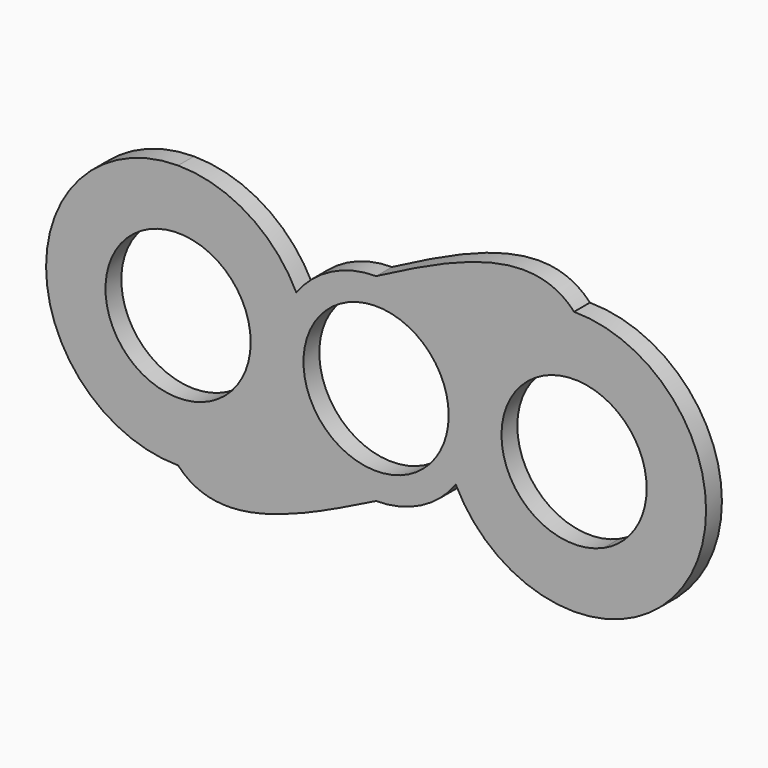
from build123d import *

# Parameters (mm, degrees)
F0_R     = 11
F1_DEPTH = 3


with BuildPart() as f1:
    # F0 (on Front) → F1 (new body)
    with BuildSketch(Plane.XZ):
        with BuildLine():
            ThreePointArc((34.4457053252, 10.0615955075), (39.2169072518, 6.0040503586), (41, -2e-10))
            ThreePointArc((41, -2e-10), (39.218122302, -6.0021847046), (34.4497779591, -10.0597950337))
            add(Edge.make_bspline(
                [(34.4497779591, -10.0597950337), (33.5572864984, -14.2139641421), (32.0732731389, -17.7845741491), (30, -20)],
                knots=[0.5781750695, 0.5781750695, 0.5781750695, 0.5781750695, 0.6822186894, 0.6822186894, 0.6822186894, 0.6822186894], degree=3))
            ThreePointArc((30, -20), (50, 0), (30, 20))
            add(Edge.make_bspline(
                [(30, 20), (32.0727475467, 17.7685869814), (33.5539058525, 14.2021827738), (34.4457053252, 10.0615955075)],
                knots=[0.3177813106, 0.3177813106, 0.3177813106, 0.3177813106, 0.4213364669, 0.4213364669, 0.4213364669, 0.4213364669], degree=3))
        make_face()
        with BuildLine():
            ThreePointArc((34.4497779591, -10.0597950337), (19.0000002253, -0.0022264354), (34.4457053252, 10.0615955075))
            add(Edge.make_bspline(
                [(30, 20), (32.0727475467, 17.7685869814), (33.5539058525, 14.2021827738), (34.4457053252, 10.0615955075)],
                knots=[0.3177813106, 0.3177813106, 0.3177813106, 0.3177813106, 0.4213364669, 0.4213364669, 0.4213364669, 0.4213364669], degree=3))
            add(Edge.make_bspline(
                [(0, 15), (11.7076504976, 21.1235117167), (23.6393275279, 26.8475716609), (30, 20)],
                knots=[0, 0, 0, 0, 0.3177813106, 0.3177813106, 0.3177813106, 0.3177813106], degree=3))
            ThreePointArc((0, 15), (-6.7706330465, 13.3850113242), (-12.0833333333, 8.8878037532))
            ThreePointArc((-12.0833333333, 8.8878037532), (-19.4585597536, 16.9964124901), (-30, 20))
            add(Edge.make_bspline(
                [(-30, 20), (-32.0727475467, 17.7685869814), (-33.5539058525, 14.2021827738), (-34.4457053252, 10.0615955075)],
                knots=[0.3177813106, 0.3177813106, 0.3177813106, 0.3177813106, 0.4213364669, 0.4213364669, 0.4213364669, 0.4213364669], degree=3))
            ThreePointArc((-34.4457053252, 10.0615955075), (-23.9959496412, 9.2169072516), (-19, -2e-10))
            ThreePointArc((-19, -2e-10), (-23.9978152957, -9.2181223023), (-34.4497779591, -10.0597950337))
            add(Edge.make_bspline(
                [(-34.4497779591, -10.0597950337), (-33.5572864984, -14.2139641421), (-32.0732731389, -17.7845741491), (-30, -20)],
                knots=[0.5781750695, 0.5781750695, 0.5781750695, 0.5781750695, 0.6822186894, 0.6822186894, 0.6822186894, 0.6822186894], degree=3))
            add(Edge.make_bspline(
                [(-30, -20), (-23.6675842682, -26.7665939655), (-11.8380817304, -20.8909455716), (0, -15)],
                knots=[0.6822186894, 0.6822186894, 0.6822186894, 0.6822186894, 1, 1, 1, 1], degree=3))
            ThreePointArc((0, -15), (6.7706330465, -13.3850113242), (12.0833333333, -8.8878037532))
            ThreePointArc((12.0833333333, -8.8878037532), (19.4585597536, -16.9964124901), (30, -20))
            add(Edge.make_bspline(
                [(34.4497779591, -10.0597950337), (33.5572864984, -14.2139641421), (32.0732731389, -17.7845741491), (30, -20)],
                knots=[0.5781750695, 0.5781750695, 0.5781750695, 0.5781750695, 0.6822186894, 0.6822186894, 0.6822186894, 0.6822186894], degree=3))
        make_face()
        Circle(F0_R, mode=Mode.SUBTRACT)
        with BuildLine():
            add(Edge.make_bspline(
                [(-30, 20), (-32.0727475467, 17.7685869814), (-33.5539058525, 14.2021827738), (-34.4457053252, 10.0615955075)],
                knots=[0.3177813106, 0.3177813106, 0.3177813106, 0.3177813106, 0.4213364669, 0.4213364669, 0.4213364669, 0.4213364669], degree=3))
            ThreePointArc((-30, 20), (-50, 0), (-30, -20))
            add(Edge.make_bspline(
                [(-34.4497779591, -10.0597950337), (-33.5572864984, -14.2139641421), (-32.0732731389, -17.7845741491), (-30, -20)],
                knots=[0.5781750695, 0.5781750695, 0.5781750695, 0.5781750695, 0.6822186894, 0.6822186894, 0.6822186894, 0.6822186894], degree=3))
            ThreePointArc((-34.4497779591, -10.0597950337), (-40.9999997747, 0.0022264349), (-34.4457053252, 10.0615955075))
        make_face()
    extrude(amount=F1_DEPTH)


solid = f1.part
